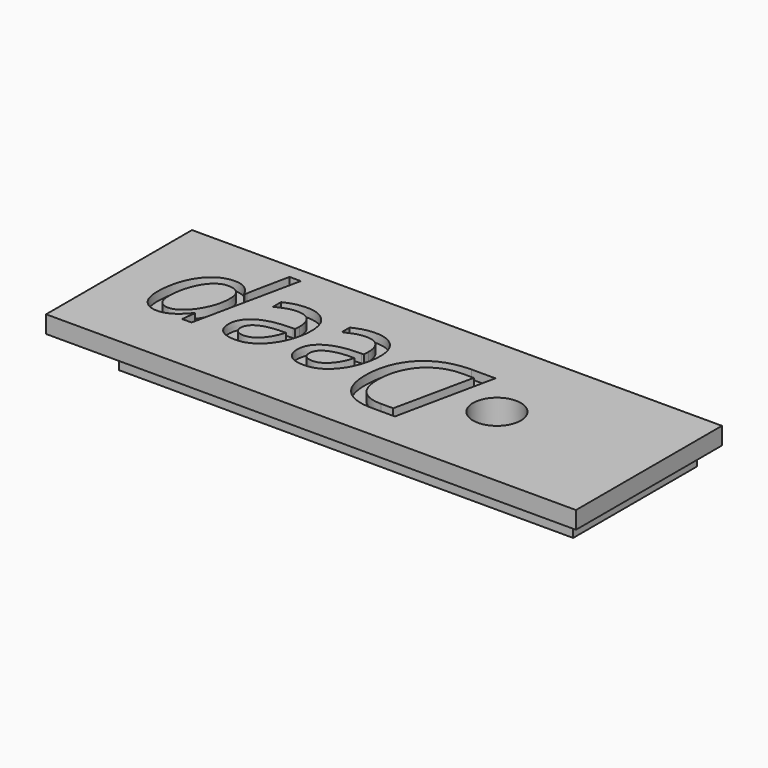
from build123d import *

# Parameters (mm, degrees)
F0_W         = 52.3
F0_H         = 17.8
F1_DEPTH     = 2
F2_W         = 52.3
F2_H         = 17.8
F3_DEPTH     = 2
F4_R         = 2.75
F5_DEPTH     = 4
F6_TEXT_SIZE = 16.0356347439
F7_DEPTH     = 1


# Not quite as in the source:
# - Text() gives the source's letters only with a copy of the font that has no kerning and outlines rounded to 1/6400 em; it was checked with that copy


with BuildPart() as f1:
    # F0 (on Top) → F1 (new body)
    with BuildSketch(Plane.XY):
        Rectangle(F0_W, F0_H)
    extrude(amount=F1_DEPTH)

    # F2 (on face) → F3 (join)
    with BuildSketch(Plane.XY.offset(2)):
        Polygon((22.0899866074, 10.5), (-33.25, 10.5), (-33.25, -10.5), (27.75, -10.5), (27.75, 10.5), (23.5818685144, 10.5), align=None)
        Rectangle(F2_W, F2_H, mode=Mode.SUBTRACT)
        Rectangle(F2_W, F2_H)
    extrude(amount=F3_DEPTH)

    # F4 (on face) → F5 (cut, through all)
    with BuildSketch(Plane.XY.offset(4)):
        with Locations((10.25, 0)):
            Circle(F4_R)
    extrude(amount=-F5_DEPTH, mode=Mode.SUBTRACT)

    # F6 (on face) → F7 (cut)
    with BuildSketch(Plane.XY.offset(4)):
        with Locations(Location((6.75, 5), (0, 0, 180))):
            Text('Deep', F6_TEXT_SIZE, font='Open Sans', font_style=FontStyle.ITALIC, text_align=(TextAlign.LEFT, TextAlign.BOTTOM))
    extrude(amount=-F7_DEPTH, mode=Mode.SUBTRACT)


solid = f1.part
